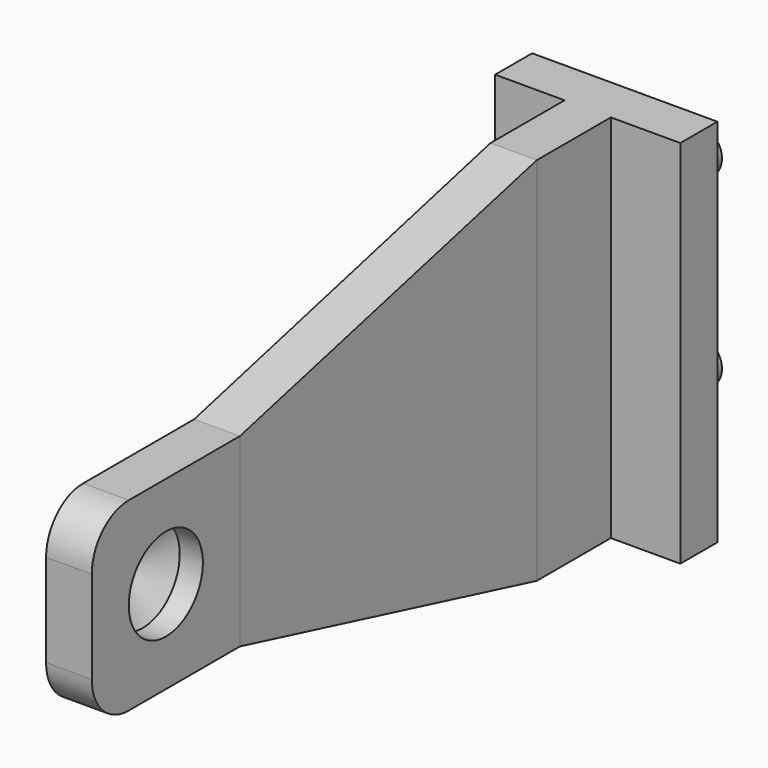
from build123d import *

# Parameters (mm, degrees)
F0_W         = 25.4
F0_H         = 50.8
F1_DEPTH     = 6.35
F2_W         = 6.35
F2_H         = 50.8
F3_DEPTH     = 12.7
F3_FACE_W    = 6.35
F3_FACE_H    = 50.8
F5_W         = 6.2655590393
F5_H         = 25.4
F7_DEPTH     = 25.4
F8_T1_DEPTH  = 38.0155590393
F10_D        = 12.7
F10_DEPTH    = 3.175
F10_TIP      = 3.8154649308
F11_T        = 4.445
F11_T3_DEPTH = 59.69
F11_T5_DEPTH = 15.1555590393
F11_T7_DEPTH = 34.29
F12_R        = 3.175
F13_DEPTH    = 12.7


# Not quite as in the source:
# - a fillet or chamfer that OpenCascade refuses, or shapes differently, is made with other operations: its cross-section is extruded or revolved along the edge and cut away or added
# - a shell that OpenCascade refuses in one call is made with other operations: the cavity is built on its own and cut out


with BuildPart() as f1:
    # F0 (on Front) → F1 (new body)
    with BuildSketch(Plane.XZ):
        with Locations((-6.5905367956, 12.3420813114)):
            Rectangle(F0_W, F0_H)
    extrude(amount=F1_DEPTH)

    # F2 (on face) → F3 (join)
    with BuildSketch(Plane.XZ.offset(6.35)):
        with Locations((-6.5905367956, 12.3420813114)):
            Rectangle(F2_W, F2_H)
    extrude(amount=F3_DEPTH)

    # F3_face (on face) → F6 section 0
    with BuildSketch(Plane(origin=(-6.5905367956, -19.05, 12.3420813114), x_dir=(1, 0, 0), z_dir=(0, -1, 0))):
        Rectangle(F3_FACE_W, F3_FACE_H)
    # F5 (on offset) → F6 section 1
    with BuildSketch(Plane.XZ.offset(69.85)):
        with Locations((-6.6327572759, 12.3420813114)):
            Rectangle(F5_W, F5_H)
    loft()

    # F7 (add): a face of the model
    f7_faces = [f1.faces().sort_by_distance(p)[0] for p in [
        (-6.6327572759, -69.85, 12.3420813114),
    ]]
    extrude(f7_faces, amount=F7_DEPTH)

    # F8: fillet of radius 6.35 on 4 edges, made by hand

    # F8_s2 → F8_t1 (cut)
    with BuildSketch(Plane.YZ.offset(-25.6405367956)):
        with BuildLine():
            ThreePointArc((-88.9, 25.0420813114), (-93.3901280605, 23.1822093719), (-95.25, 18.6920813114))
            Line((-95.25, 18.6920813114), (-95.25, 25.0420813114))
            Line((-95.25, 25.0420813114), (-88.9, 25.0420813114))
        make_face()
        with BuildLine():
            ThreePointArc((-88.9, -0.3579186886), (-93.3901280605, 1.5019532508), (-95.25, 5.9920813114))
            Line((-95.25, 5.9920813114), (-95.25, -0.3579186886))
            Line((-95.25, -0.3579186886), (-88.9, -0.3579186886))
        make_face()
    extrude(amount=F8_T1_DEPTH, mode=Mode.SUBTRACT)

    # F10
    with Locations(Plane.YZ.offset(-3.4999777563)):
        with Locations((-82.55, 12.3420813114)):
            Hole(F10_D / 2, depth=F10_DEPTH)
            with Locations((0, 0, -(F10_DEPTH + F10_TIP / 2))):  # 118° drill point
                Cone(0, F10_D / 2, F10_TIP, mode=Mode.SUBTRACT)

    # F11: shell of thickness 4.445, made by hand


with BuildPart() as f11_core1:
    # F11_t2: copy of F1
    add(f1.part)

    # the walls: a layer under each face that stays
    f11_faces = [f11_core1.faces().sort_by_distance(p)[0] for p in [
        (-19.2905367956, -3.175, 12.3420813114),
        (-6.5905367956, -9.525, 37.7420813114),
        (-6.5905367956, -9.525, -13.0579186886),
        (-6.5905367956, 0, 12.3420813114),
        (-14.5280367956, -6.35, 12.3420813114),
        (6.1094632044, -3.175, 12.3420813114),
        (1.3469632044, -6.35, 12.3420813114),
        (-3.4155367956, -12.7, 12.3420813114),
        (-6.6116470357, -44.45, 31.3920813114),
        (-6.6116470357, -44.45, -6.7079186886),
        (-3.4577572759, -44.45, 12.3420813114),
        (-6.6327572759, -79.375, 25.0420813114),
        (-6.6327572759, -79.375, -0.3579186886),
        (-6.6327572759, -93.3901280605, 23.1822093719),
        (-6.6327572759, -93.3901280606, 1.5019532508),
        (-6.6327572759, -95.25, 12.3420813114),
        (-8.2202572759, -86.328223001, 12.3420813114),
        (-3.4999777563, -91.0166666667, 3.8754146447),
        (-5.0874777563, -88.9, 12.3420813114),
    ]]
    thicken(f11_faces, amount=-F11_T, mode=Mode.SUBTRACT)

    # F11_s4 → F11_t3 (cut)
    with BuildSketch(Plane.XY.offset(-17.5029186886)):
        Polygon((-3.3710867956, -6.39445), (-3.4155367956, -1.905), (-7.8605367956, -1.905), (-7.8605367956, -6.35), align=None)
    extrude(amount=F11_T3_DEPTH, mode=Mode.SUBTRACT)

    # F11_s6 → F11_t5 (cut)
    with BuildSketch(Plane.YZ.offset(-14.2105367956)):
        Polygon((-69.8607807085, 25.1296541455), (-68.7719291467, 20.7297978982), (-69.3027954941, 20.5970813114), (-69.85, 20.5970813114), align=None)
        Polygon((-69.8607807085, -0.4454915228), (-68.7719291467, 3.9543647245), (-69.3027954941, 4.0870813114), (-69.85, 4.0870813114), align=None)
    extrude(amount=F11_T5_DEPTH, mode=Mode.SUBTRACT)

    # F11_s8 → F11_t7 (cut)
    with BuildSketch(Plane.XY.offset(-4.8029186886)):
        Polygon((-3.4110778177, -69.8500738857), (-7.9449716156, -69.8426114261), (-7.9449777563, -69.8463057105), (-7.9449777563, -69.85), align=None)
    extrude(amount=F11_T7_DEPTH, mode=Mode.SUBTRACT)

    # F11_s9 → F11_t10 (revolve, cut)
    with BuildSketch(Plane.XY.offset(12.3420813114)):
        Polygon((-6.6368766698, -76.2673434424), (-10.4850864079, -73.910655757), (-9.1898377553, -71.755), (-6.6749777563, -71.755), align=None)
    revolve(axis=Axis((-6.6749777563, -82.55, 12.3420813114), (1, 0, 0)), mode=Mode.SUBTRACT)


with BuildPart() as f1_1:
    add(f1.part)

    # what is left inside the walls is the cavity
    f11_cavity = [f11_core1.part.solids().sort_by_distance(p)[0] for p in [
        (-9.721087, -28.696773, 12.342081),
        (-9.611738, -89.747742, 5.14434),
        (-9.611738, -89.747742, 19.539823),
    ]]
    add(f11_cavity, mode=Mode.SUBTRACT)

    # F12 (on face) → F13 (join)
    with BuildSketch(Plane(origin=(0, 0, 0), x_dir=(-1, 0, 0), z_dir=(0, 1, 0))):
        with Locations((6.5905367956, 25.0420813114)):
            Circle(F12_R)
        with Locations((6.5905367956, -0.3579186886)):
            Circle(F12_R)
    extrude(amount=F13_DEPTH)


solid = f1_1.part
